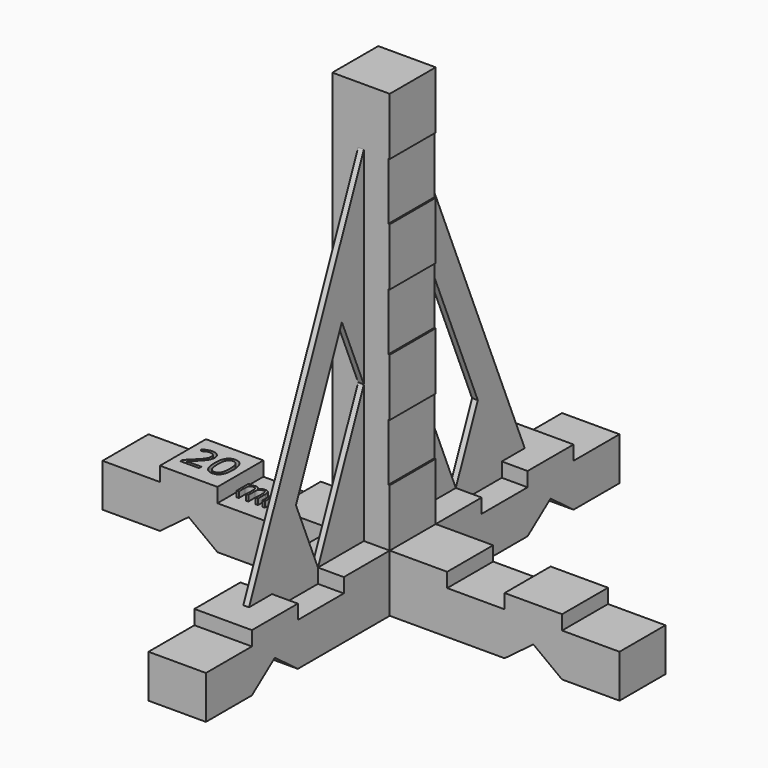
from build123d import *

# Parameters (mm, degrees)
F0_W          = 20
F0_H          = 20
F1_DEPTH      = 160
F2_W          = 20
F2_H          = 20
F3_DEPTH      = 80
F3_DEPTH_BACK = 100
F4_W          = 20
F4_H          = 20
F5_DEPTH      = 80
F5_DEPTH_BACK = 100
F6_W          = 20
F6_H          = 5
F6_W_2        = 0.5
F6_H_2        = 20
F7_DEPTH      = 25
F8_W          = 20
F8_H          = 5
F9_DEPTH      = 25
F12_DEPTH     = 1
F14_DEPTH     = 25
F16_DEPTH     = 25
F18_DEPTH     = 25
F19_TEXT_SIZE = 13.809844909
F21_DEPTH     = 3
F20_TEXT_SIZE = 9.7610574479
F22_DEPTH     = 2


# Not quite as in the source:
# - Text() gives the source's letters only with a copy of the font that has no kerning and outlines rounded to 1/6400 em; it was checked with that copy


with BuildPart() as f1:
    # F0 (on Top) → F1 (new body)
    with BuildSketch(Plane.XY):
        with Locations((10, -10)):
            Rectangle(F0_W, F0_H)
    extrude(amount=F1_DEPTH)

    # F2 (on face) → F3 (join, two sides)
    with BuildSketch(Plane.YZ.offset(20)) as f3_sk:
        with Locations((-10, 10)):
            Rectangle(F2_W, F2_H)
    extrude(amount=F3_DEPTH)
    extrude(f3_sk.sketch, amount=-F3_DEPTH_BACK)

    # F4 (on face) → F5 (join, two sides)
    with BuildSketch(Plane.XZ.offset(20)) as f5_sk:
        with Locations((10, 10)):
            Rectangle(F4_W, F4_H)
    extrude(amount=F5_DEPTH)
    extrude(f5_sk.sketch, amount=-F5_DEPTH_BACK)

    # F6 (on face) → F7 (cut)
    with BuildSketch(Plane.XZ.offset(20)):
        with Locations((-70, 17.5)):
            Rectangle(F6_W, F6_H)
        with Locations((-30, 17.5)):
            Rectangle(F6_W, F6_H)
        with Locations((50, 17.5)):
            Rectangle(F6_W, F6_H)
        with Locations((90, 17.5)):
            Rectangle(F6_W, F6_H)
        with Locations((19.75, 50)):
            Rectangle(F6_W_2, F6_H_2)
        with Locations((19.75, 90)):
            Rectangle(F6_W_2, F6_H_2)
        with Locations((19.75, 130)):
            Rectangle(F6_W_2, F6_H_2)
    extrude(amount=-F7_DEPTH, mode=Mode.SUBTRACT)

    # F8 (on face) → F9 (cut)
    with BuildSketch(Plane.YZ.offset(20)):
        with Locations((-90, 17.5)):
            Rectangle(F8_W, F8_H)
        with Locations((-50, 17.5)):
            Rectangle(F8_W, F8_H)
        with Locations((30, 17.5)):
            Rectangle(F8_W, F8_H)
        with Locations((70, 17.5)):
            Rectangle(F8_W, F8_H)
    extrude(amount=-F9_DEPTH, mode=Mode.SUBTRACT)

    # F11 (on offset) → F12 (join, symmetric)
    with BuildSketch(Plane(origin=(10, 0, 0), x_dir=(0, -1, 0), z_dir=(-1, 0, 0))):
        Polygon((0, 20), (0, 140), (-50, 20), (-40, 20), (-30, 44), (-20, 20), (-7.8928291587, 20), align=None)
        Polygon((-7.8928291587, 97.057210019), (-7.8928291587, 20), (-23.9464145794, 58.5286050095), align=None, mode=Mode.SUBTRACT)
        Polygon((70, 20), (20, 140), (20, 20), (28.3242450259, 20), (40, 20), (50, 44), (60, 20), align=None)
        Polygon((44.1621225129, 58.010905969), (28.3242450259, 20), (28.3242450259, 96.0218119379), align=None, mode=Mode.SUBTRACT)
        Polygon((-23.9464145794, 58.5286050095), (-7.8928291587, 20), (-7.8928291587, 97.057210019), align=None)
        Polygon((28.3242450259, 96.0218119379), (28.3242450259, 20), (44.1621225129, 58.010905969), align=None)
        Polygon((60, 15), (60, 20), (50, 44), (40, 20), (40, 15), align=None)
        Polygon((-30, 44), (-40, 20), (-40, 15), (-20, 15), (-20, 20), align=None)
    extrude(amount=F12_DEPTH, both=True)

    # F13 (on face) → F14 (cut)
    with BuildSketch(Plane(origin=(0, 0, 0), x_dir=(-1, 0, 0), z_dir=(0, 1, 0))):
        Polygon((-70, 7.5), (-80, 0), (-60, 0), align=None)
        Polygon((40, 0), (60, 0), (50, 7.5), align=None)
    extrude(amount=-F14_DEPTH, mode=Mode.SUBTRACT)

    # F15 (on face) → F16 (cut)
    with BuildSketch(Plane(origin=(0, 0, 0), x_dir=(0, -1, 0), z_dir=(-1, 0, 0))):
        Polygon((-50, 7.5), (-60, 0), (-40, 0), align=None)
        Polygon((60, 0), (80, 0), (70, 7.5), align=None)
    extrude(amount=-F16_DEPTH, mode=Mode.SUBTRACT)

    # F17 (on face) → F18 (cut)
    with BuildSketch(Plane(origin=(9, 0, 0), x_dir=(0, -1, 0), z_dir=(-1, 0, 0))):
        Polygon((-29.5833333333, 43), (-20, 20), (0, 68), (-9.5833333333, 91), align=None)
        Polygon((49.5833333333, 43), (29.5833333333, 91), (20, 68), (40, 20), align=None)
    extrude(amount=-F18_DEPTH, mode=Mode.SUBTRACT)

    # F19 (on face) → F21 (cut)
    with BuildSketch(Plane.XY.offset(20)):
        with Locations((-58, -14.4743120932)):
            Text('20', F19_TEXT_SIZE, font='Open Sans', text_align=(TextAlign.LEFT, TextAlign.BOTTOM))
    extrude(amount=-F21_DEPTH, mode=Mode.SUBTRACT)

    # F20 (on face) → F22 (join)
    with BuildSketch(Plane.XY.offset(15)):
        with Locations((-39, -14)):
            Text('mm', F20_TEXT_SIZE, font='Open Sans', text_align=(TextAlign.LEFT, TextAlign.BOTTOM))
    extrude(amount=F22_DEPTH)


solid = f1.part
